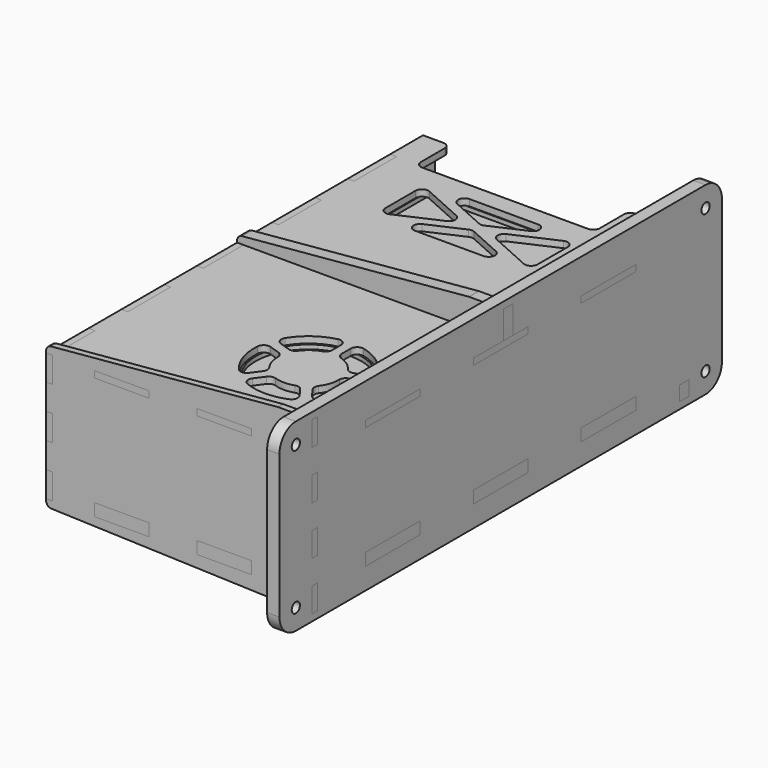
from build123d import *

# Parameters (mm, degrees)
F2_W           = 115
F2_H           = 216
F3_DEPTH       = 51
F4_R           = 24.5
F4_W           = 70
F4_H           = 31
F5_DEPTH       = 2
F4_W_2         = 110
F4_H_2         = 20
F6_DEPTH       = 25
F7_W           = 23
F7_H           = 152
F8_DEPTH       = 2
F9_D           = 3.5
F9_DEPTH       = 6.35
F9_TIP         = 1.0515060833
F10_W          = 257.1
F10_H          = 85.725
F11_DEPTH      = 5.715
F12_W          = 5.715
F12_H          = 11.3392857143
F13_DEPTH      = 2.9972
F14_R          = 1.75
F14_W          = 25.4
F14_H          = 2.9972
F15_DEPTH      = 5.715
F17_DEPTH      = 2.9972
F19_DEPTH      = 2.9972
F24_DEPTH      = 5.715
F26_DEPTH      = 5.715
F29_R          = 2
F29_R_2        = 1.75
F29_W          = 17.681875
F29_H          = 31.2690625
F29_H_2        = 33.2690625
F29_W_2        = 14.824375
F30_DEPTH      = 75.766
F31_R          = 5.715
F32_W          = 83.25
F32_H          = 20
F33_DEPTH      = 69.6732
F34_F1_R       = 2.9972
F34_F2_R       = 2.9972
F34_2_T1_DEPTH = 3.6700339255
F34_3_T1_DEPTH = 6.3878339255
F35_R          = 9.525
F37_D          = 4.7625
F38_R          = 2.54
F38_2_R        = 2.54
F38_3_R        = 2.54


# Not quite as in the source:
# - a fillet or chamfer that OpenCascade refuses, or shapes differently, is made with other operations: its cross-section is extruded or revolved along the edge and cut away or added


with BuildPart() as f3:
    # F2 (on Top) → F3 (new body)
    with BuildSketch(Plane.XY):
        Rectangle(F2_W, F2_H)
    extrude(amount=F3_DEPTH)

    # F4 (on face) → F5 (cut)
    with BuildSketch(Plane.XY.offset(51)):
        with Locations((21.5, -61)):
            Circle(F4_R)
        with Locations((0, 63.5)):
            Rectangle(F4_W, F4_H)
    extrude(amount=-F5_DEPTH, mode=Mode.SUBTRACT)

    # F4 (on face) → F6 (cut)
    with BuildSketch(Plane.XY.offset(51)):
        with Locations((0, 98)):
            Rectangle(F4_W_2, F4_H_2)
    extrude(amount=-F6_DEPTH, mode=Mode.SUBTRACT)

    # F7 (on face) → F8 (cut)
    with BuildSketch(Plane(origin=(0, 0, 0), x_dir=(1, 0, 0), z_dir=(0, 0, -1))):
        with Locations((46, 1)):
            Rectangle(F7_W, F7_H)
        with Locations((-46, 1)):
            Rectangle(F7_W, F7_H)
    extrude(amount=-F8_DEPTH, mode=Mode.SUBTRACT)

    # F9
    with Locations(Plane(origin=(0, 0, 0), x_dir=(1, 0, 0), z_dir=(0, 0, -1))):
        with Locations((25.5, 74.5), (-25.5, 74.5), (25.5, -75.5), (-25.5, -75.5)):
            Hole(F9_D / 2, depth=F9_DEPTH)
            with Locations((0, 0, -(F9_DEPTH + F9_TIP / 2))):  # 118° drill point
                Cone(0, F9_D / 2, F9_TIP, mode=Mode.SUBTRACT)


with BuildPart() as f11:
    # F10 (on face) → F11 (new body)
    with BuildSketch(Plane.YZ.offset(57.5)):
        with Locations((-1.5, 27.1875)):
            Rectangle(F10_W, F10_H)
    extrude(amount=F11_DEPTH)


with BuildPart() as f13:
    # F12 (on face) → F13 (new body)
    with BuildSketch(Plane.XZ.offset(108)):
        Polygon((47.34, -12.5), (63.215, -12.5), (63.215, -1.1607142857), (57.5, -1.1607142857), (57.5, 0), (-57.5, 0), (-57.5, 51), (57.5, 51), (57.5, 55.5357142857), (63.215, 55.5357142857), (63.215, 66.875), (47.34, 66.875), (-60.4972, 57.1722), (-60.4972, -8.89), align=None)
        Polygon((57.5, 0), (57.5, 10.1785714286), (57.5, 21.5178571429), (57.5, 32.8571428571), (57.5, 44.1964285714), (57.5, 51), (-57.5, 51), (-57.5, 0), align=None)
        with Locations((60.3575, 38.5267857143)):
            Rectangle(F12_W, F12_H)
        with Locations((60.3575, 15.8482142857)):
            Rectangle(F12_W, F12_H)
    extrude(amount=F13_DEPTH)


with BuildPart() as f15:
    # F14 (on face) → F15 (new body)
    with BuildSketch(Plane(origin=(0, 0, 0), x_dir=(1, 0, 0), z_dir=(0, 0, -1))):
        Polygon((-60.4972, -108), (-57.5, -108), (-57.5, -75), (-34.5, -75), (-34.5, 77), (-57.5, 77), (-57.5, 108), (-60.4972, 108), align=None)
        Polygon((57.5, -108), (57.5, -77.0632), (57.5, -75), (34.5, -75), (34.5, 77), (57.5, 77), (57.5, 80.0604), (57.5, 108), (35.1009333333, 108), (9.7009333333, 108), (-12.6981333333, 108), (-38.0981333333, 108), (-57.5, 108), (-57.5, 77), (-34.5, 77), (-34.5, -75), (-57.5, -75), (-57.5, -108), align=None)
        with Locations((-25.5, -75.5)):
            Circle(F14_R, mode=Mode.SUBTRACT)
        with Locations((25.5, -75.5)):
            Circle(F14_R, mode=Mode.SUBTRACT)
        with Locations((-25.5, 74.5)):
            Circle(F14_R, mode=Mode.SUBTRACT)
        with Locations((25.5, 74.5)):
            Circle(F14_R, mode=Mode.SUBTRACT)
        with Locations((22.4009333333, 109.4986)):
            Rectangle(F14_W, F14_H)
        with Locations((-25.3981333333, 109.4986)):
            Rectangle(F14_W, F14_H)
        Polygon((57.5, -77.0632), (63.215, -77.0632), (63.215, -45.3132), (57.5, -45.3132), (57.5, -14.3764), (63.215, -14.3764), (63.215, 17.3736), (57.5, 17.3736), (57.5, 48.3104), (63.215, 48.3104), (63.215, 80.0604), (57.5, 80.0604), (57.5, 77), (34.5, 77), (34.5, -75), (57.5, -75), align=None)
    extrude(amount=F15_DEPTH)


with BuildPart() as f17:
    # F16 (on face) → F17 (new body)
    with BuildSketch(Plane.XY.offset(51)):
        Polygon((57.5, 108), (-60.4972, 108), (-60.4972, -108), (-38.0981333333, -108), (-38.0981333333, -110.9972), (-12.6981333333, -110.9972), (-12.6981333333, -108), (9.7009333333, -108), (9.7009333333, -110.9972), (35.1009333333, -110.9972), (35.1009333333, -108), (57.5, -108), (57.5, -80.0604), (63.215, -80.0604), (63.215, -48.3104), (57.5, -48.3104), (57.5, -17.3736), (63.215, -17.3736), (63.215, 14.3764), (57.5, 14.3764), (57.5, 45.3132), (63.215, 45.3132), (63.215, 77.0632), (57.5, 77.0632), align=None)
    extrude(amount=F17_DEPTH)


with BuildPart() as f19:
    # F18 (on face) → F19 (new body)
    with BuildSketch(Plane(origin=(-57.5, 0, 0), x_dir=(0, -1, 0), z_dir=(-1, 0, 0))):
        Polygon((-64.20056, 53.9972), (-88.95, 53.9972), (-88.95, 51), (-108, 51), (-108, 0), (-88.95, 0), (-88.95, -5.715), (-64.20056, -5.715), (-64.20056, 0), (-45.15056, 0), (-45.15056, -5.715), (-20.40112, -5.715), (-20.40112, 0), (-1.35112, 0), (-1.35112, -5.715), (23.39832, -5.715), (23.39832, 0), (42.44832, 0), (42.44832, -5.715), (67.19776, -5.715), (67.19776, 0), (86.24776, 0), (86.24776, -5.715), (110.9972, -5.715), (110.9972, 6.22744), (108, 6.22744), (108, 18.16988), (110.9972, 18.16988), (110.9972, 30.11232), (108, 30.11232), (108, 42.05476), (110.9972, 42.05476), (110.9972, 53.9972), (86.24776, 53.9972), (86.24776, 51), (67.19776, 51), (67.19776, 53.9972), (42.44832, 53.9972), (42.44832, 51), (23.39832, 51), (23.39832, 53.9972), (-1.35112, 53.9972), (-1.35112, 51), (-20.40112, 51), (-20.40112, 53.9972), (-45.15056, 53.9972), (-45.15056, 51), (-64.20056, 51), align=None)
    extrude(amount=F19_DEPTH)


with BuildPart() as f17_1:
    add(f17.part)

    # F20: cut F19
    add(f19.part, mode=Mode.SUBTRACT)


with BuildPart() as f15_1:
    add(f15.part)

    # F20: cut F19
    add(f19.part, mode=Mode.SUBTRACT)


with BuildPart() as f11_1:
    add(f11.part)

    # F20: cut F19
    add(f19.part, mode=Mode.SUBTRACT)


with BuildPart() as f13_1:
    add(f13.part)

    # F21: cut F17, F19, F15
    add(f17_1.part, mode=Mode.SUBTRACT)
    add(f19.part, mode=Mode.SUBTRACT)
    add(f15_1.part, mode=Mode.SUBTRACT)


with BuildPart() as f11_2:
    add(f11_1.part)

    # F22: cut F17, F13, F15
    add(f17_1.part, mode=Mode.SUBTRACT)
    add(f13_1.part, mode=Mode.SUBTRACT)
    add(f15_1.part, mode=Mode.SUBTRACT)


with BuildPart() as f24:
    # F23 (on face) → F24 (new body)
    with BuildSketch(Plane(origin=(0, 108, 0), x_dir=(-1, 0, 0), z_dir=(0, 1, 0))):
        Polygon((-47.34, -12.5), (60.4972, -8.89), (60.4972, -5.715), (34.925, -5.715), (34.925, 0), (22.225, 0), (22.225, -5.715), (-22.225, -5.715), (-22.225, 0), (-34.925, 0), (-34.925, -5.715), (-63.215, -5.715), (-63.215, -12.5), align=None)
    extrude(amount=-F24_DEPTH)


with BuildPart() as f26:
    # F25 (on Front) → F26 (new body)
    with BuildSketch(Plane.XZ):
        Polygon((63.215, 66.875), (47.34, 66.875), (-60.4972, 57.1722), (-60.4972, 53.9972), (-34.925, 53.9972), (-34.925, 51), (-22.225, 51), (-22.225, 53.9972), (22.225, 53.9972), (22.225, 51), (34.925, 51), (34.925, 53.9972), (57.5, 53.9972), (63.215, 53.9972), align=None)
    extrude(amount=-F26_DEPTH)


with BuildPart() as f11_3:
    add(f11_2.part)

    # F27: cut F26
    add(f26.part, mode=Mode.SUBTRACT)

    # F28: cut F24
    add(f24.part, mode=Mode.SUBTRACT)

    # F35
    f35_edges = [f11_3.edges().sort_by_distance(p)[0] for p in [
        (60.3575, 127.05, 70.05),
        (60.3575, 127.05, -15.675),
        (60.3575, -130.05, 70.05),
        (60.3575, -130.05, -15.675),
    ]]
    fillet(f35_edges, radius=F35_R)

    # F37 (through all)
    with Locations(Plane(origin=(57.5, 0, 0), x_dir=(0, -1, 0), z_dir=(-1, 0, 0))):
        with Locations((-117.525, 60.525), (-117.525, -6.15), (120.525, 60.525), (120.525, -6.15)):
            Hole(F37_D / 2)


with BuildPart() as f17_2:
    add(f17_1.part)

    # F27: cut F26
    add(f26.part, mode=Mode.SUBTRACT)

    # F32 (on face) → F33 (cut, through all)
    with BuildSketch(Plane.XY.offset(53.9972)):
        Polygon((-5.4869013869, 63.5), (-35.396875, 76.9326861278), (-35.396875, 50.0673138722), align=None)
        Polygon((29.9099736131, 79.396875), (-29.9099736131, 79.396875), (0, 65.9641888722), align=None)
        Polygon((35.396875, 76.9326861278), (5.4869013869, 63.5), (35.396875, 50.0673138722), align=None)
        Polygon((29.9099736131, 47.603125), (0, 61.0358111278), (-29.9099736131, 47.603125), align=None)
        with BuildLine():
            ThreePointArc((38.1270537893, -80.0608203221), (44.5253591812, -71.4693182032), (46.79375, -61))
            ThreePointArc((46.79375, -61), (46.6336151336, -58.1583139903), (46.1552381638, -55.3526094391))
            Line((46.1552381638, -55.3526094391), (35.6136255331, -58.7777870129))
            ThreePointArc((35.6136255331, -58.7777870129), (35.7439650564, -59.8854975448), (35.7875, -61))
            ThreePointArc((35.7875, -61), (34.7024155858, -66.4615820921), (31.6119788873, -71.0935890165))
            Line((31.6119788873, -71.0935890165), (38.1270537893, -80.0608203221))
        make_face()
        with BuildLine():
            Line((34.2243469298, -54.5020271269), (44.7659595605, -51.0768495532))
            ThreePointArc((44.7659595605, -51.0768495532), (36.3672932252, -40.5369263985), (23.7479, -35.8063354263))
            Line((23.7479, -35.8063354263), (23.7479, -46.89044289))
            ThreePointArc((23.7479, -46.89044289), (29.8979817921, -49.4411696929), (34.2243469298, -54.5020271269))
        make_face()
        with BuildLine():
            ThreePointArc((8.7756530702, -54.5020271269), (13.1020182079, -49.4411696929), (19.2521, -46.89044289))
            Line((19.2521, -46.89044289), (19.2521, -35.8063354263))
            ThreePointArc((19.2521, -35.8063354263), (6.6327067748, -40.5369263985), (-1.7659595605, -51.0768495532))
            Line((-1.7659595605, -51.0768495532), (8.7756530702, -54.5020271269))
        make_face()
        with BuildLine():
            Line((4.8729462107, -80.0608203221), (11.3880211127, -71.0935890165))
            ThreePointArc((11.3880211127, -71.0935890165), (7.9117800234, -65.4150803071), (7.3863744669, -58.7777870129))
            Line((7.3863744669, -58.7777870129), (-3.1552381638, -55.3526094391))
            ThreePointArc((-3.1552381638, -55.3526094391), (-2.555785759, -68.8161986015), (4.8729462107, -80.0608203221))
        make_face()
        with BuildLine():
            ThreePointArc((8.510124814, -82.7033852593), (21.5, -86.29375), (34.489875186, -82.7033852593))
            Line((34.489875186, -82.7033852593), (27.974800284, -73.7361539537))
            ThreePointArc((27.974800284, -73.7361539537), (21.5, -75.2875), (15.025199716, -73.7361539537))
            Line((15.025199716, -73.7361539537), (8.510124814, -82.7033852593))
        make_face()
        with Locations((-6.35, 98)):
            Rectangle(F32_W, F32_H)
    extrude(amount=-F33_DEPTH, mode=Mode.SUBTRACT)

    # F34: fillet of radius 2.9972 on 36 edges, made by hand

    # F34_f1
    f34_f1_edges = [f17_2.edges().sort_by_distance(p)[0] for p in [
        (35.275, 88, 52.4986),
        (-47.975, 88, 52.4986),
        (-35.396875, 50.0673138722, 52.4986),
        (5.4869013869, 63.5, 52.4986),
        (-29.9099736131, 47.603125, 52.4986),
        (0, 61.0358111278, 52.4986),
        (-5.4869013869, 63.5, 52.4986),
        (0, 65.9641888722, 52.4986),
        (-35.396875, 76.9326861278, 52.4986),
        (-29.9099736131, 79.396875, 52.4986),
        (29.9099736131, 79.396875, 52.4986),
        (35.396875, 76.9326861278, 52.4986),
        (35.396875, 50.0673138722, 52.4986),
        (29.9099736131, 47.603125, 52.4986),
        (8.510124814, -82.7033852593, 52.4986),
        (4.8729462107, -80.0608203221, 52.4986),
        (15.025199716, -73.7361539537, 52.4986),
        (11.3880211127, -71.0935890165, 52.4986),
        (7.3863744669, -58.7777870129, 52.4986),
        (-3.1552381638, -55.3526094391, 52.4986),
        (8.7756530702, -54.5020271269, 52.4986),
        (-1.7659595605, -51.0768495532, 52.4986),
        (19.2521, -35.8063354263, 52.4986),
        (19.2521, -46.89044289, 52.4986),
        (23.7479, -46.89044289, 52.4986),
        (23.7479, -35.8063354263, 52.4986),
        (34.2243469298, -54.5020271269, 52.4986),
        (44.7659595605, -51.0768495532, 52.4986),
        (46.1552381638, -55.3526094391, 52.4986),
        (35.6136255331, -58.7777870129, 52.4986),
        (31.6119788873, -71.0935890165, 52.4986),
        (38.1270537893, -80.0608203221, 52.4986),
        (34.489875186, -82.7033852593, 52.4986),
        (27.974800284, -73.7361539537, 52.4986),
    ]]
    fillet(f34_f1_edges, radius=F34_F1_R)

    # F34_f2
    f34_f2_edges = [f17_2.edges().sort_by_distance(p)[0] for p in [
        (35.275, 108, 52.4986),
        (-47.975, 108, 52.4986),
    ]]
    fillet(f34_f2_edges, radius=F34_F2_R)


with BuildPart() as f15_2:
    add(f15_1.part)

    # F28: cut F24
    add(f24.part, mode=Mode.SUBTRACT)

    # F29 (on face) → F30 (cut, through all)
    with BuildSketch(Plane(origin=(0, 0, -5.715), x_dir=(1, 0, 0), z_dir=(0, 0, -1))):
        with Locations((-25.5, -75.5)):
            Circle(F29_R)
        with Locations((-25.5, -75.5)):
            Circle(F29_R_2, mode=Mode.SUBTRACT)
        with Locations((25.5, -75.5)):
            Circle(F29_R)
        with Locations((25.5, -75.5)):
            Circle(F29_R_2, mode=Mode.SUBTRACT)
        with Locations((-25.5, 74.5)):
            Circle(F29_R)
        with Locations((-25.5, 74.5)):
            Circle(F29_R_2, mode=Mode.SUBTRACT)
        with Locations((25.5, 74.5)):
            Circle(F29_R)
        with Locations((25.5, 74.5)):
            Circle(F29_R_2, mode=Mode.SUBTRACT)
        with Locations((-42.9440625, -59.76234375)):
            Rectangle(F29_W, F29_H)
        with Locations((-42.9440625, 60.76234375)):
            Rectangle(F29_W, F29_H_2)
        with Locations((41.5153125, -59.76234375)):
            Rectangle(F29_W_2, F29_H)
        with Locations((41.5153125, 60.76234375)):
            Rectangle(F29_W_2, F29_H_2)
        with Locations((-42.9440625, -19.92078125)):
            Rectangle(F29_W, F29_H)
        with Locations((-42.9440625, 19.92078125)):
            Rectangle(F29_W, F29_H)
        with Locations((41.5153125, -19.92078125)):
            Rectangle(F29_W_2, F29_H)
        with Locations((41.5153125, 19.92078125)):
            Rectangle(F29_W_2, F29_H)
    extrude(amount=-F30_DEPTH, mode=Mode.SUBTRACT)

    # F31
    f31_edges = [f15_2.edges().sort_by_distance(p)[0] for p in [
        (48.9275, -44.127813, -2.8575),
        (48.9275, -4.28625, -2.8575),
        (48.9275, 35.555313, -2.8575),
        (48.9275, 75.396875, -2.8575),
        (-34.103125, 75.396875, -2.8575),
        (-34.103125, 35.555313, -2.8575),
        (-34.103125, -4.28625, -2.8575),
        (-34.103125, -44.127813, -2.8575),
        (48.9275, 44.127813, -2.8575),
        (48.9275, 4.28625, -2.8575),
        (48.9275, -35.555313, -2.8575),
        (48.9275, -77.396875, -2.8575),
        (-34.103125, -77.396875, -2.8575),
        (-34.103125, -35.555313, -2.8575),
        (-34.103125, 4.28625, -2.8575),
        (-34.103125, 44.127813, -2.8575),
        (34.103125, 44.127813, -2.8575),
        (34.103125, 4.28625, -2.8575),
        (34.103125, -35.555313, -2.8575),
        (34.103125, -77.396875, -2.8575),
        (-51.785, -77.396875, -2.8575),
        (-51.785, -35.555313, -2.8575),
        (-51.785, 4.28625, -2.8575),
        (-51.785, 44.127813, -2.8575),
        (34.103125, -44.127813, -2.8575),
        (34.103125, -4.28625, -2.8575),
        (34.103125, 35.555313, -2.8575),
        (34.103125, 75.396875, -2.8575),
        (-51.785, 75.396875, -2.8575),
        (-51.785, 35.555313, -2.8575),
        (-51.785, -4.28625, -2.8575),
        (-51.785, -44.127813, -2.8575),
    ]]
    fillet(f31_edges, radius=F31_R)


with BuildPart() as f13_2:
    add(f13_1.part)

    # F34#2: fillet of radius 2.9972 on 1 edges, made by hand

    # F34_2_s2 → F34_2_t1 (cut)
    with BuildSketch(Plane.XZ.offset(107.6635830373)):
        with BuildLine():
            ThreePointArc((47.4745667851, 66.875), (47.3401354242, 66.8719837033), (47.205974639, 66.8629408843))
            Line((47.205974639, 66.8629408843), (47.34, 66.875))
            Line((47.34, 66.875), (47.4745667851, 66.875))
        make_face()
    extrude(amount=F34_2_T1_DEPTH, mode=Mode.SUBTRACT)

    # F38
    f38_edges = [f13_2.edges().sort_by_distance(p)[0] for p in [
        (-60.4972, -109.4986, -8.89),
        (-60.4972, -109.4986, 57.1722),
        (47.34, -109.4986, -12.5),
    ]]
    fillet(f38_edges, radius=F38_R)


with BuildPart() as f26_1:
    add(f26.part)

    # F34#3: fillet of radius 2.9972 on 1 edges, made by hand

    # F34_3_s2 → F34_3_t1 (cut)
    with BuildSketch(Plane.XZ.offset(-6.0514169627)):
        with BuildLine():
            ThreePointArc((47.4745667851, 66.875), (47.3401354242, 66.8719837033), (47.205974639, 66.8629408843))
            Line((47.205974639, 66.8629408843), (47.34, 66.875))
            Line((47.34, 66.875), (47.4745667851, 66.875))
        make_face()
    extrude(amount=F34_3_T1_DEPTH, mode=Mode.SUBTRACT)

    # F38#3
    f38_3_edges = [f26_1.edges().sort_by_distance(p)[0] for p in [
        (-60.4972, 2.8575, 57.1722),
    ]]
    fillet(f38_3_edges, radius=F38_3_R)


with BuildPart() as f24_1:
    add(f24.part)

    # F38#2
    f38_2_edges = [f24_1.edges().sort_by_distance(p)[0] for p in [
        (-60.4972, 105.1425, -8.89),
        (47.34, 105.1425, -12.5),
    ]]
    fillet(f38_2_edges, radius=F38_2_R)


solid = Compound([f3.part, f19.part, f11_3.part, f17_2.part, f15_2.part, f13_2.part, f26_1.part, f24_1.part])
